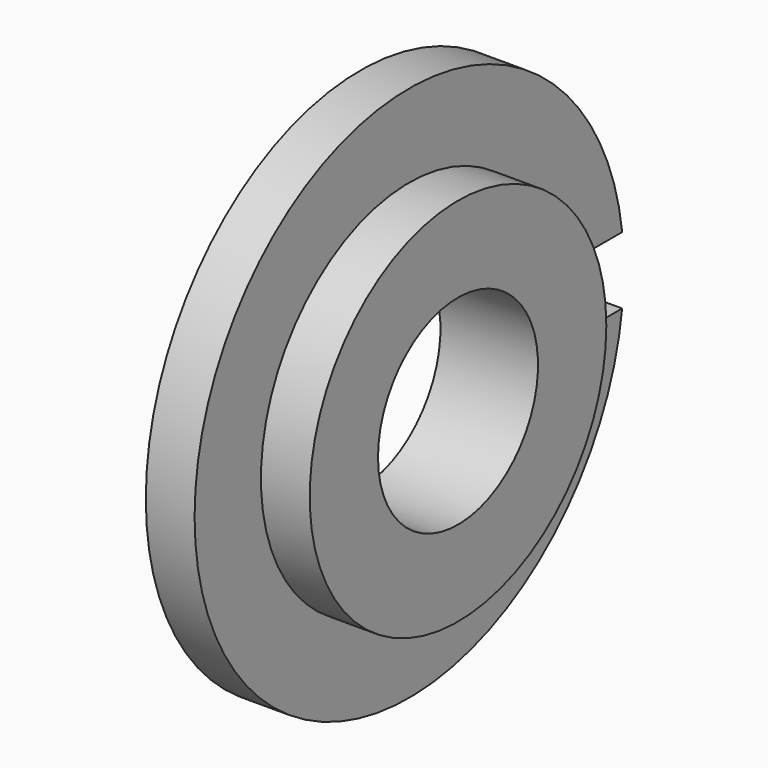
from build123d import *

# Parameters (mm, degrees)
F0_R     = 11
F0_R_2   = 7.6
F1_DEPTH = 2
F2_DEPTH = 2
F3_R     = 4.1
F4_DEPTH = 25
F6_DEPTH = 5


# Not quite as in the source:
# - a feature names something its author has since deleted; it is built from what else it names


with BuildPart() as f1:
    # F0 (on Right) → F1 (new body)
    with BuildSketch(Plane.YZ):
        Circle(F0_R)
        Circle(F0_R_2, mode=Mode.SUBTRACT)
        Circle(F0_R_2)
    extrude(amount=-F1_DEPTH)

    # F0 (on Right) → F2 (join)
    with BuildSketch(Plane.YZ):
        Circle(F0_R_2)
    extrude(amount=F2_DEPTH)

    # F3 (on face) → F4 (cut)
    with BuildSketch(Plane(origin=(-2, 0, 0), x_dir=(0, -1, 0), z_dir=(-1, 0, 0))):
        Circle(F3_R)
    extrude(amount=-F4_DEPTH, mode=Mode.SUBTRACT)

    # F5 (on face) → F6 (cut)
    with BuildSketch(Plane(origin=(-2, 0, 0), x_dir=(0, -1, 0), z_dir=(-1, 0, 0))):
        with BuildLine():
            ThreePointArc((-10.9129812948, -1.3808835065), (-10.9999996004, -0.0029651094), (-10.9137241581, 1.375))
            Line((-10.9137241581, 1.375), (-11.6283151001, 1.375))
            Line((-11.6283151001, 1.375), (-11.6283151001, -1.3808835065))
            Line((-11.6283151001, -1.3808835065), (-10.9129812948, -1.3808835065))
        make_face()
        with BuildLine():
            Line((-9.6, -1.375), (-9.6, 1.375))
            ThreePointArc((-9.6, 1.375), (-10.975, 0), (-9.6, -1.375))
        make_face()
        with BuildLine():
            ThreePointArc((-9.6, -1.375), (-10.975, 0), (-9.6, 1.375))
            Line((-9.6, 1.375), (-10.9137241581, 1.375))
            ThreePointArc((-10.9137241581, 1.375), (-10.9999996004, -0.0029651094), (-10.9129812948, -1.3808835065))
            Line((-10.9129812948, -1.3808835065), (-9.6, -1.3808835065))
            Line((-9.6, -1.3808835065), (-9.6, -1.375))
        make_face()
        with BuildLine():
            ThreePointArc((-9.6, -1.375), (-8.6277281759, -0.9722718241), (-8.225, 0))
            ThreePointArc((-8.225, 0), (-8.6277281759, 0.9722718241), (-9.6, 1.375))
            Line((-9.6, 1.375), (-9.6, -1.375))
        make_face()
    extrude(amount=-F6_DEPTH, mode=Mode.SUBTRACT)


solid = f1.part
